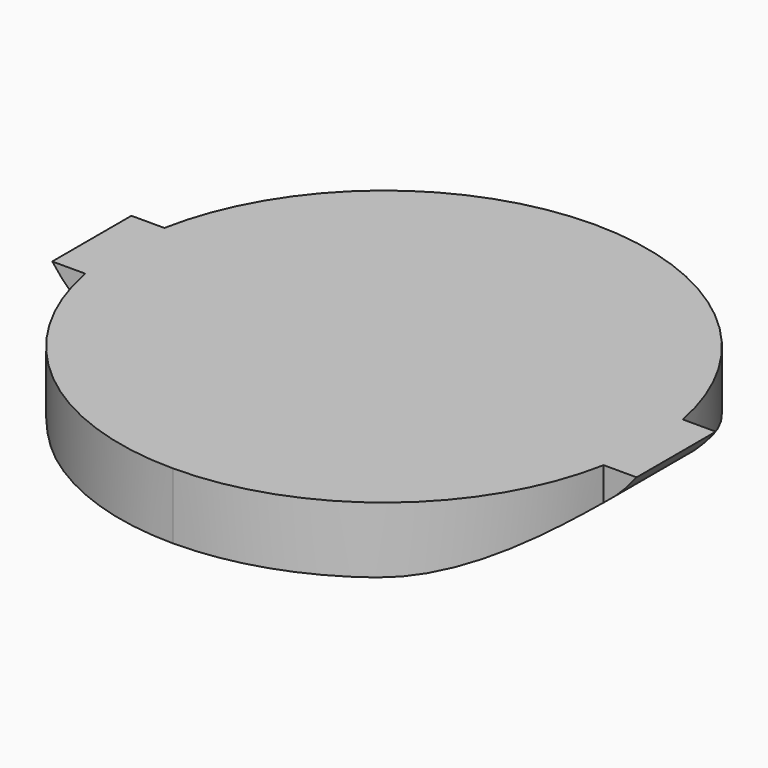
from build123d import *

# Parameters (mm, degrees)
F1_DEPTH    = 2
F2_T1_DEPTH = 23


# Not quite as in the source:
# - a fillet or chamfer that OpenCascade refuses, or shapes differently, is made with other operations: its cross-section is extruded or revolved along the edge and cut away or added


with BuildPart() as f1:
    # F0 (on Top) → F1 (new body)
    with BuildSketch(Plane.XY):
        with BuildLine():
            Line((0, 0), (8, 0))
            ThreePointArc((8, 0), (7.964450219, 0.7533476681), (7.8581168228, 1.5))
            ThreePointArc((7.8581168228, 1.5), (5.0990195136, 6.164414003), (0, 8))
            Line((0, 8), (0, 0))
        make_face()
        with BuildLine():
            Line((8.8581168228, 0), (8, 0))
            ThreePointArc((8, 0), (7.964450219, -0.7533476681), (7.8581168228, -1.5))
            Line((7.8581168228, -1.5), (8.8581168228, -1.5))
            Line((8.8581168228, -1.5), (8.8581168228, 0))
        make_face()
        with BuildLine():
            ThreePointArc((7.8581168228, 1.5), (7.964450219, 0.7533476681), (8, 0))
            Line((8, 0), (8.8581168228, 0))
            Line((8.8581168228, 0), (8.8581168228, 1.5))
            Line((8.8581168228, 1.5), (7.8581168228, 1.5))
        make_face()
        with BuildLine():
            ThreePointArc((7.8581168228, -1.5), (7.964450219, -0.7533476681), (8, 0))
            Line((8, 0), (0, 0))
            Line((0, 0), (0, -8))
            ThreePointArc((0, -8), (5.0990195136, -6.164414003), (7.8581168228, -1.5))
        make_face()
        with BuildLine():
            Line((-8, 0), (0, 0))
            Line((0, 0), (0, 8))
            ThreePointArc((0, 8), (-5.0990195136, 6.164414003), (-7.8581168228, 1.5))
            ThreePointArc((-7.8581168228, 1.5), (-7.964450219, 0.7533476681), (-8, 0))
        make_face()
        with BuildLine():
            Line((0, -8), (0, 0))
            Line((0, 0), (-8, 0))
            ThreePointArc((-8, 0), (-7.964450219, -0.7533476681), (-7.8581168228, -1.5))
            ThreePointArc((-7.8581168228, -1.5), (-5.0990195136, -6.164414003), (0, -8))
        make_face()
        with BuildLine():
            Line((-8.8581168228, 0), (-8, 0))
            ThreePointArc((-8, 0), (-7.964450219, 0.7533476681), (-7.8581168228, 1.5))
            Line((-7.8581168228, 1.5), (-8.8581168228, 1.5))
            Line((-8.8581168228, 1.5), (-8.8581168228, 0))
        make_face()
        with BuildLine():
            ThreePointArc((-7.8581168228, -1.5), (-7.964450219, -0.7533476681), (-8, 0))
            Line((-8, 0), (-8.8581168228, 0))
            Line((-8.8581168228, 0), (-8.8581168228, -1.5))
            Line((-8.8581168228, -1.5), (-7.8581168228, -1.5))
        make_face()
    extrude(amount=F1_DEPTH)

    # F2: fillet of radius 5 on 2 edges, made by hand

    # F2_s2 → F2_t1 (cut)
    with BuildSketch(Plane.XZ.offset(-11.5)):
        with BuildLine():
            ThreePointArc((-8.8581168228, 2), (-7.0941848003, 0.527864045), (-4.8581168228, 0))
            Line((-4.8581168228, 0), (-8.8581168228, 0))
            Line((-8.8581168228, 0), (-8.8581168228, 2))
        make_face()
        with BuildLine():
            ThreePointArc((8.8581168228, 2), (7.0941848003, 0.527864045), (4.8581168228, 0))
            Line((4.8581168228, 0), (8.8581168228, 0))
            Line((8.8581168228, 0), (8.8581168228, 2))
        make_face()
    extrude(amount=F2_T1_DEPTH, mode=Mode.SUBTRACT)


solid = f1.part
